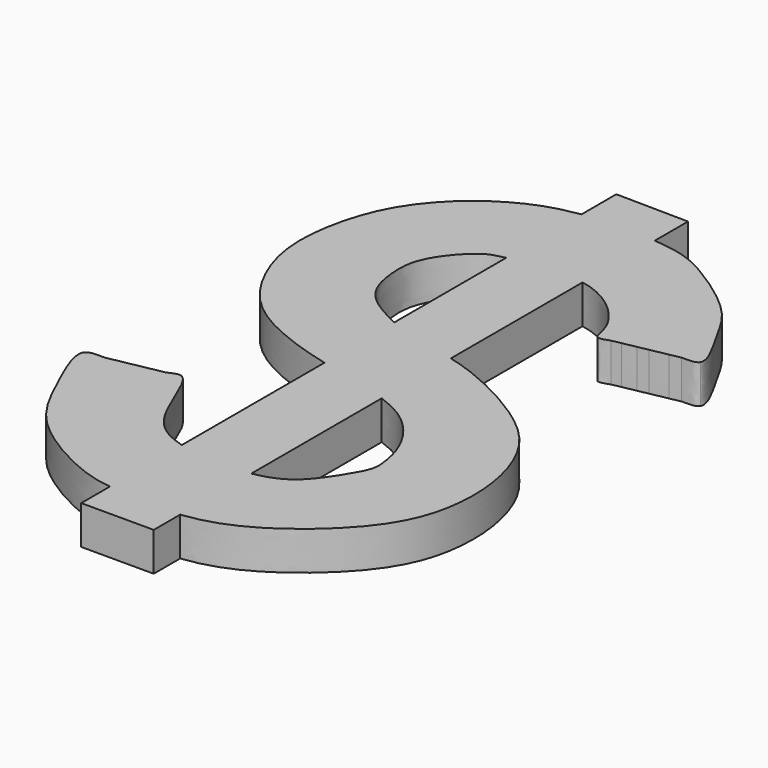
from build123d import *

# Parameters (mm, degrees)
F1_DEPTH = 5
F3_DEPTH = 5


# Not quite as in the source:
# - ends of sketch curves that miss each other by under 0.0002 mm in the source are joined


with BuildPart() as f1:
    # F0 (on Top) → F1 (new body)
    with BuildSketch(Plane.XY):
        with BuildLine():
            add(Edge.make_bspline(
                [(35.4062364212, 26.4075431064), (36.1136138051, 26.4375571122), (37.1920857039, 26.3162993106), (37.5000004827, 26.8173329532)],
                knots=[0.9891130914, 0.9891130914, 0.9891130914, 0.9891130914, 1, 1, 1, 1], degree=3))
            Line((37.5000004827, 26.8173329532), (35.4062364212, 26.4075431064))
        make_face()
        with BuildLine():
            Line((35.4062364212, 26.4075431064), (37.5000004827, 26.8173329532))
            add(Edge.make_bspline(
                [(37.5000004827, 26.8173329532), (37.9973083609, 27.626543796), (34.9123021991, 32.5873489734), (32.7949088716, 37.1897556584), (24.3027338054, 43.1267309099), (19.169003707, 44.8923617288), (7.4598902451, 45.1060959203), (1.1897145625, 42.6781312373), (-3.8120923938, 39.3082420584), (-8.3975827588, 33.8837589271), (-10.6150276555, 26.8781022613), (-11.0693390019, 19.8953460452), (-8.6400083438, 13.0680757921), (-3.8097449962, 6.818918491), (7.098891731, 2.7978051401), (18.6539113372, 0.7987680613), (23.4954239403, -3.2235491862), (25.6191120408, -7.1395973632), (26.1759914014, -9.9044108084), (26.4578971493, -12.1962753352), (24.05257382, -15.9975311089), (20.2331488923, -21.4307798521), (6.3264948767, -20.8637776593), (1.7512699941, -16.0141911602), (-0.3644556238, -8.9908558965), (-1.4762532664, -8.344146423)],
                knots=[0, 0, 0, 0, 0.0175832594, 0.0358597298, 0.0588860231, 0.0769168699, 0.1019008471, 0.1213566894, 0.1392971613, 0.1589566475, 0.1790587295, 0.1986072677, 0.2183003743, 0.2387106394, 0.2641094999, 0.2897108509, 0.3079044406, 0.3232934463, 0.3355975298, 0.3464371002, 0.3617101189, 0.3803717423, 0.4066458723, 0.4263882219, 0.4468914028, 0.4468914028, 0.4468914028, 0.4468914028], degree=3))
            Line((-1.4762532664, -8.344146423), (-3.3538070747, -8.7043670617))
            add(Edge.make_bspline(
                [(-3.3538070747, -8.7043670617), (-4.3961030163, -9.0785878191), (-5.7923316991, -9.172210662), (-6.977947746, -9.3996772122)],
                knots=[0.4571971679, 0.4571971679, 0.4571971679, 0.4571971679, 0.4714944637, 0.4714944637, 0.4714944637, 0.4714944637], degree=3))
            add(Edge.make_bspline(
                [(-6.977947746, -9.3996772122), (-6.9813423589, -9.4003284862), (-8.0810994233, -9.6117855626), (-8.9980666521, -9.939542333), (-10.0812918203, -9.9950777943)],
                knots=[0.4714944637, 0.4714944637, 0.4714944637, 0.4714944637, 0.4715353992, 0.4847631381, 0.4847631381, 0.4847631381, 0.4847631381], degree=3))
            Line((-10.0812918203, -9.9950777943), (-12.4999995173, -10.459122248))
            add(Edge.make_bspline(
                [(-12.4999995173, -10.459122248), (-13.126901554, -11.4363217572), (-10.0620076243, -18.071207169), (-6.6572928739, -25.453264179), (3.6944606077, -31.1633139716), (8.9573246108, -31.9190126967), (19.2131315433, -32.828607643), (28.1944728773, -27.9884701152), (35.3339415951, -20.9026515006), (37.9212850063, -14.0402369382), (37.8967425581, -6.45170622), (35.5823181115, 0.3428764855), (30.8312502632, 5.7611625668), (19.729691585, 11.6834204472), (11.6697951489, 12.6692531996), (7.461612409, 14.3735968882), (2.0146611718, 17.3677263892), (0.8400309809, 22.2167360632), (0.8804248433, 26.9117301401), (5.0986415272, 31.7191380502), (7.7382723724, 32.3960622929), (18.908113489, 34.7526975815), (25.7548504177, 27.5466796426), (25.5917068321, 24.7768521377), (26.0184388608, 24.57017079)],
                knots=[0.4964601716, 0.4964601716, 0.4964601716, 0.4964601716, 0.5162392615, 0.5388537913, 0.5634156905, 0.5809728234, 0.6041261586, 0.627965304, 0.6513159606, 0.6711925222, 0.6914715047, 0.7110009296, 0.7308632035, 0.7572517914, 0.778353885, 0.7941959907, 0.8121364664, 0.8281945183, 0.8442785556, 0.8621343822, 0.874711514, 0.8989580497, 0.9214301919, 0.9329361544, 0.9329361544, 0.9329361544, 0.9329361544], degree=3))
            Line((26.0184388608, 24.57017079), (27.4935914991, 24.8588864981))
            add(Edge.make_bspline(
                [(27.493591499, 24.8588864981), (27.9377033488, 24.9991084414), (28.2605398181, 25.0247596569), (28.689210115, 25.0928920283)],
                knots=[0.9420743235, 0.9420743235, 0.9420743235, 0.9420743235, 0.9503012391, 0.9503012391, 0.9503012391, 0.9503012391], degree=3))
            Line((28.689210115, 25.0928920283), (30.3940653973, 25.4265649563))
            add(Edge.make_bspline(
                [(30.3940653973, 25.4265649563), (30.8684922538, 25.525339568), (31.2367282875, 25.5988500193), (31.7592196718, 25.6937518716)],
                knots=[0.9601251512, 0.9601251512, 0.9601251512, 0.9601251512, 0.9689160154, 0.9689160154, 0.9689160154, 0.9689160154], degree=3))
            Line((31.7592196718, 25.6937518716), (33.9809155123, 26.128580425))
            add(Edge.make_bspline(
                [(33.9809155123, 26.128580425), (34.49158124, 26.255037971), (34.8225983305, 26.3827793559), (35.4062364212, 26.4075431064)],
                knots=[0.9801305953, 0.9801305953, 0.9801305953, 0.9801305953, 0.9891130914, 0.9891130914, 0.9891130914, 0.9891130914], degree=3))
        make_face()
        with BuildLine():
            Line((33.9809155123, 26.128580425), (35.4062364212, 26.4075431064))
            add(Edge.make_bspline(
                [(33.9809155123, 26.128580425), (34.49158124, 26.255037971), (34.8225983305, 26.3827793559), (35.4062364212, 26.4075431064)],
                knots=[0.9801305953, 0.9801305953, 0.9801305953, 0.9801305953, 0.9891130914, 0.9891130914, 0.9891130914, 0.9891130914], degree=3))
        make_face()
        with BuildLine():
            Line((-3.3538070747, -8.7043670617), (-1.4762532664, -8.344146423))
            add(Edge.make_bspline(
                [(-1.4762532664, -8.344146423), (-2.0350897385, -8.0190829163), (-2.6025001683, -8.434621562), (-3.3538070747, -8.7043670617)],
                knots=[0.4468914028, 0.4468914028, 0.4468914028, 0.4468914028, 0.4571971679, 0.4571971679, 0.4571971679, 0.4571971679], degree=3))
        make_face()
        with BuildLine():
            add(Edge.make_bspline(
                [(31.7592196718, 25.6937518716), (32.4257663489, 25.8148189671), (33.3433531298, 25.9706991145), (33.9809155123, 26.128580425)],
                knots=[0.9689160154, 0.9689160154, 0.9689160154, 0.9689160154, 0.9801305953, 0.9801305953, 0.9801305953, 0.9801305953], degree=3))
            Line((33.9809155123, 26.128580425), (31.7592196718, 25.6937518716))
        make_face()
        with BuildLine():
            add(Edge.make_bspline(
                [(-3.3538070747, -8.7043670617), (-4.3961030163, -9.0785878191), (-5.7923316991, -9.172210662), (-6.977947746, -9.3996772122)],
                knots=[0.4571971679, 0.4571971679, 0.4571971679, 0.4571971679, 0.4714944637, 0.4714944637, 0.4714944637, 0.4714944637], degree=3))
            Line((-3.3538070747, -8.7043670617), (-6.977947746, -9.3996772122))
        make_face()
        with BuildLine():
            Line((30.3940653973, 25.4265649563), (31.7592196718, 25.6937518716))
            add(Edge.make_bspline(
                [(30.3940653973, 25.4265649563), (30.8684922538, 25.525339568), (31.2367282875, 25.5988500193), (31.7592196718, 25.6937518716)],
                knots=[0.9601251512, 0.9601251512, 0.9601251512, 0.9601251512, 0.9689160154, 0.9689160154, 0.9689160154, 0.9689160154], degree=3))
        make_face()
        with BuildLine():
            add(Edge.make_bspline(
                [(-6.977947746, -9.3996772122), (-6.9813423589, -9.4003284862), (-8.0810994233, -9.6117855626), (-8.9980666521, -9.939542333), (-10.0812918203, -9.9950777943)],
                knots=[0.4714944637, 0.4714944637, 0.4714944637, 0.4714944637, 0.4715353992, 0.4847631381, 0.4847631381, 0.4847631381, 0.4847631381], degree=3))
            Line((-6.977947746, -9.3996772122), (-10.0812918203, -9.9950777943))
        make_face()
        with BuildLine():
            add(Edge.make_bspline(
                [(28.689210115, 25.0928920283), (29.2010932456, 25.1742501533), (29.8638868401, 25.316182965), (30.3940653973, 25.4265649563)],
                knots=[0.9503012391, 0.9503012391, 0.9503012391, 0.9503012391, 0.9601251512, 0.9601251512, 0.9601251512, 0.9601251512], degree=3))
            Line((30.3940653973, 25.4265649563), (28.689210115, 25.0928920283))
        make_face()
        with BuildLine():
            Line((-12.4999995173, -10.459122248), (-10.0812918203, -9.9950777943))
            add(Edge.make_bspline(
                [(-10.0812918203, -9.9950777943), (-11.0391668712, -10.0441867278), (-12.129259803, -9.8812222802), (-12.4999995173, -10.459122248)],
                knots=[0.4847631381, 0.4847631381, 0.4847631381, 0.4847631381, 0.4964601716, 0.4964601716, 0.4964601716, 0.4964601716], degree=3))
        make_face()
        with BuildLine():
            Line((27.4935914991, 24.8588864981), (28.689210115, 25.0928920283))
            add(Edge.make_bspline(
                [(27.493591499, 24.8588864981), (27.9377033488, 24.9991084414), (28.2605398181, 25.0247596569), (28.689210115, 25.0928920283)],
                knots=[0.9420743235, 0.9420743235, 0.9420743235, 0.9420743235, 0.9503012391, 0.9503012391, 0.9503012391, 0.9503012391], degree=3))
        make_face()
        with BuildLine():
            add(Edge.make_bspline(
                [(26.0184388608, 24.57017079), (26.357354393, 24.4060220637), (27.0002876466, 24.7031328858), (27.493591499, 24.8588864981)],
                knots=[0.9329361544, 0.9329361544, 0.9329361544, 0.9329361544, 0.9420743235, 0.9420743235, 0.9420743235, 0.9420743235], degree=3))
            Line((27.4935914991, 24.8588864981), (26.0184388608, 24.57017079))
        make_face()
    extrude(amount=F1_DEPTH)

    # F2 (on Top) → F3 (join)
    with BuildSketch(Plane.XY):
        Polygon((17.2941591591, 50.0820688903), (7.9089542851, 50.2142570913), (7.9089542851, -36.3675840199), (17.2941591591, -36.3675840199), align=None)
    extrude(amount=F3_DEPTH)


solid = f1.part
